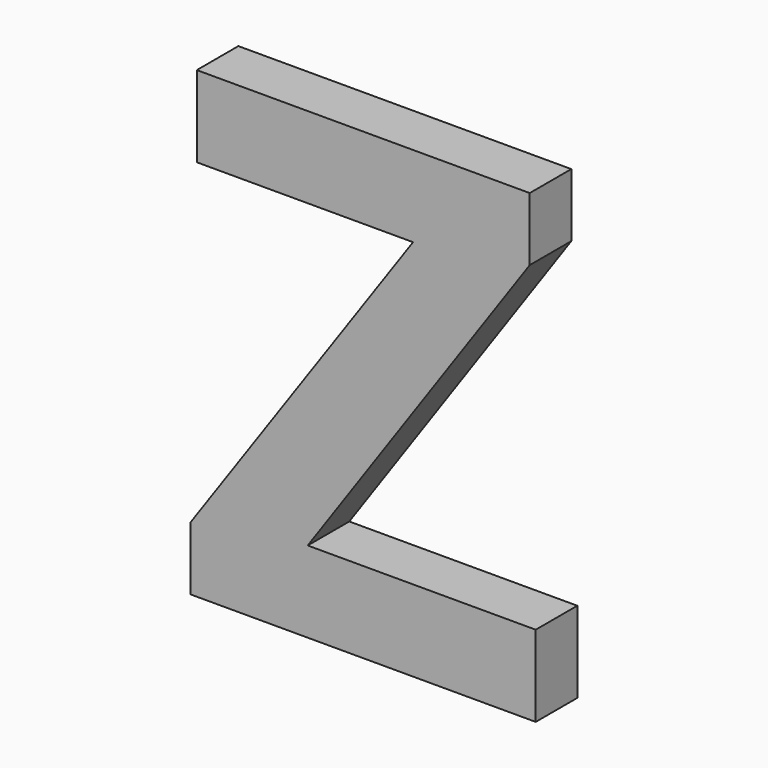
from build123d import *

# Parameters (mm, degrees)
F0_TEXT_SIZE = 62.5
F1_DEPTH     = 5


# Not quite as in the source:
# - Text() gives the source's letters only with a copy of the font that has no kerning and outlines rounded to 1/6400 em; it was checked with that copy


with BuildPart() as f1:
    # F0 (on Front) → F1 (new body)
    with BuildSketch(Plane.XZ):
        with Locations((-64.0625024117, 3.8541669409)):
            Text('Z', F0_TEXT_SIZE, font='Open Sans', font_style=FontStyle.BOLD, text_align=(TextAlign.LEFT, TextAlign.BOTTOM))
    extrude(amount=F1_DEPTH)


solid = f1.part
